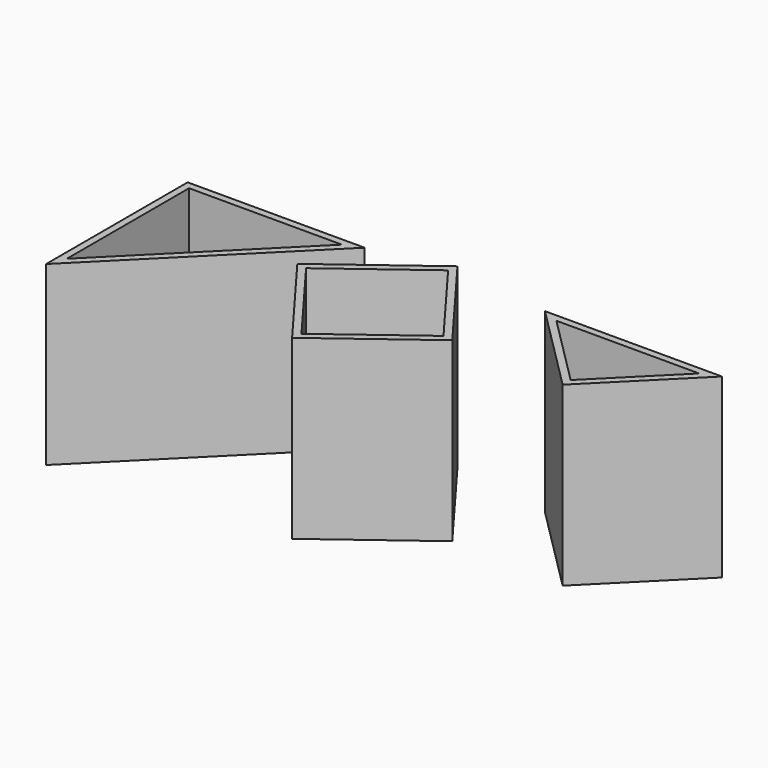
from build123d import *

# Parameters (mm, degrees)
F1_DEPTH = 50
F2_T     = -2
F2_2_T   = -2
F2_3_T   = -2


# Not quite as in the source:
# - a feature names something its author has since deleted; it is built from what else it names


with BuildPart() as f1:
    # F0 (on Top) → F1 (new body)
    with BuildSketch(Plane.XY):
        Polygon((-73.8333829338, 28.3337179901), (-123.8333829338, 28.3337179901), (-123.8333829338, -21.6662820099), align=None)
    extrude(amount=F1_DEPTH)

    # F2#3
    f2_3_openings = [f1.faces().sort_by_distance(p)[0] for p in [
        (-107.166716, 11.667051, 50),
    ]]
    offset(amount=F2_3_T, openings=f2_3_openings)


with BuildPart() as f1b:
    # F0 (on Top) → F1, piece 2 (new body)
    with BuildSketch(Plane.XY):
        Polygon((-31.1075429039, 5.8839563866), (-52.2822653136, 34.1970475437), (-80.5953564708, 13.0223251341), (-59.4206340611, -15.2907660231), align=None)
    extrude(amount=F1_DEPTH)

    # F2#2
    f2_2_openings = [f1b.faces().sort_by_distance(p)[0] for p in [
        (-55.85145, 9.453141, 50),
    ]]
    offset(amount=F2_2_T, openings=f2_2_openings)


with BuildPart() as f1c:
    # F0 (on Top) → F1, piece 3 (new body)
    with BuildSketch(Plane.XY):
        Polygon((26.1802889407, 29.5160934329), (-23.8197110593, 29.5160934329), (1.1802889407, 4.5160934329), align=None)
    extrude(amount=F1_DEPTH)

    # F2
    f2_openings = [f1c.faces().sort_by_distance(p)[0] for p in [
        (1.180289, 21.18276, 50),
    ]]
    offset(amount=F2_T, openings=f2_openings)


solid = Compound([f1.part, f1b.part, f1c.part])
